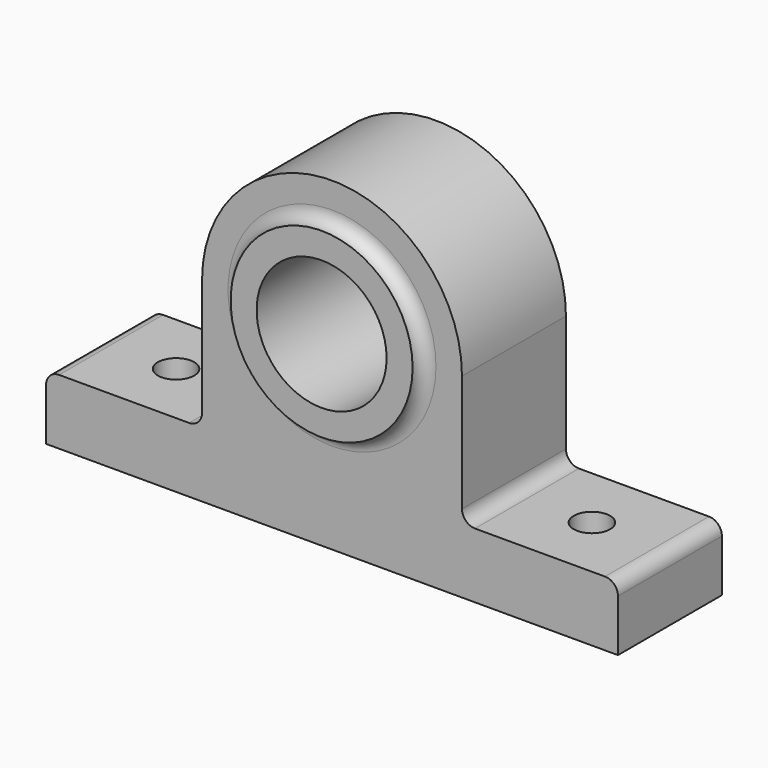
from build123d import *

# Parameters (mm, degrees)
F0_R       = 32.5
F0_R_2     = 25
F1_DEPTH   = 50
F4_D       = 14
F4_ON_F3_D = 14
F5_R       = 5
F6_R       = 35
F6_R_2     = 25
F7_DEPTH   = 50
F8_R       = 35
F8_R_2     = 25
F9_DEPTH   = 5
F10_DEPTH  = 60
F11_R      = 4.99999


# Not quite as in the source:
# - a fillet or chamfer is up to 0.001 mm smaller than in the source, because OpenCascade refuses the exact size


with BuildPart() as f1:
    # F0 (on Front) → F1 (new body)
    with BuildSketch(Plane.XZ):
        with BuildLine():
            ThreePointArc((-50, 0), (0, -50), (50, 0))
            ThreePointArc((50, 0), (0, 50), (-50, 0))
        make_face()
        Circle(F0_R, mode=Mode.SUBTRACT)
        with BuildLine():
            Line((50, -50), (50, 0))
            ThreePointArc((50, 0), (0, -50), (-50, 0))
            Line((-50, 0), (-50, -50))
            Line((-50, -50), (-110, -50))
            Line((-110, -50), (-110, -75))
            Line((-110, -75), (110, -75))
            Line((110, -75), (110, -50))
            Line((110, -50), (50, -50))
        make_face()
        Circle(F0_R)
        Circle(F0_R_2, mode=Mode.SUBTRACT)
    extrude(amount=F1_DEPTH)

    # F4 (through all)
    with Locations(Plane.XY.offset(-50)):
        with Locations((-80, -25)):
            Hole(F4_D / 2)

    # F4 on F3 (through all)
    with Locations(Plane.XY.offset(-50)):
        with Locations((80, -25)):
            Hole(F4_ON_F3_D / 2)

    # F5
    f5_edges = [f1.edges().sort_by_distance(p)[0] for p in [
        (50, -25, -50),
        (-50, -25, -50),
        (110, -25, -50),
        (-110, -25, -50),
    ]]
    fillet(f5_edges, radius=F5_R)

    # F6 (on face) → F7 (join)
    with BuildSketch(Plane(origin=(0, 0, 0), x_dir=(-1, 0, 0), z_dir=(0, 1, 0))):
        Circle(F6_R)
        Circle(F6_R_2, mode=Mode.SUBTRACT)
    extrude(amount=-F7_DEPTH)

    # F8 (on face) → F9 (join)
    with BuildSketch(Plane.XZ.offset(50)):
        Circle(F8_R)
        Circle(F8_R_2, mode=Mode.SUBTRACT)
    extrude(amount=F9_DEPTH)

    # F10 (add): a face of the model
    f10_faces = [f1.faces().sort_by_distance(p)[0] for p in [
        (-34.0100505063, -55, 0),
    ]]
    extrude(f10_faces, amount=-F10_DEPTH)

    # F11 (radius 5 in the source; OpenCascade refuses exactly that, so slightly less here)
    f11_edges = [f1.edges().sort_by_distance(p)[0] for p in [
        (-35, -50, 0),
        (-35, 0, 0),
    ]]
    fillet(f11_edges, radius=F11_R)


solid = f1.part
